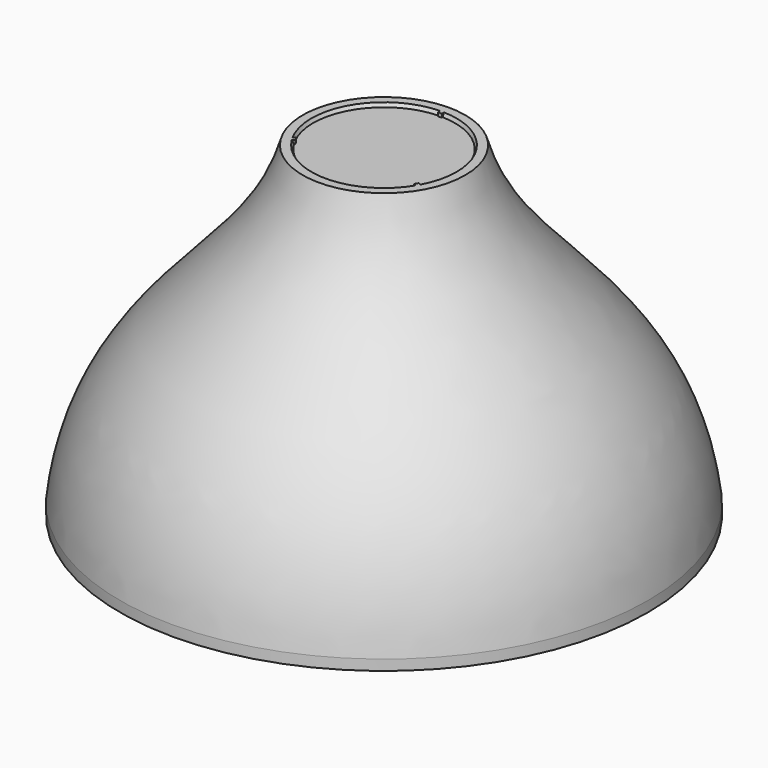
from build123d import *

# Parameters (mm, degrees)
F4_DEPTH        = 2.7018745767
F4_COPIES_COUNT = 3


# Not quite as in the source:
# - a pattern or mirror of a feature is missing from the dataset's text; its kind, count and spacing are read off the source's solid


with BuildPart() as f2:
    # F0 (on Front) → F2 (revolve)
    with BuildSketch(Plane.XZ):
        with BuildLine():
            Line((53.6962079262, 28.8167757166), (0, 28.8167757166))
            Line((0, 28.8167757166), (0, -215.1266485453))
            Line((0, -215.1266485453), (200, -215.1266485453))
            Line((200, -215.1266485453), (200, -212.5729433804))
            Line((200, -212.5729433804), (200, -207.1854621172))
            add(Edge.make_bspline(
                [(61.6075841476, 31.5186502934), (87.6578390598, -62.1243081987), (185.5585724115, -83.8800296187), (200, -207.1854621172)],
                knots=[0, 0, 0, 0, 275.9204850082, 275.9204850082, 275.9204850082, 275.9204850082], degree=3))
            Line((61.6075841476, 31.5186502934), (59, 31.5186502934))
            Line((59, 31.5186502934), (57, 31.5186502934))
            Line((57, 31.5186502934), (55, 31.5186502934))
            Line((55, 31.5186502934), (53.6962079262, 28.8167757166))
        make_face()
    revolve(axis=Axis((0, 0, -61.6418045454), (0, 0, -1)))

    # F3 (on face) → F4 (join, through all)
    with BuildSketch(Plane.XY.offset(31.5186502934)):
        Polygon((-1.5, 52.8230071068), (0, 52.8230071068), (1.5, 52.8230071068), (1.5, 55.3230071068), (0, 55.3230071068), (-1.5, 55.3230071068), align=None)
    f4 = extrude(amount=-F4_DEPTH)

    # F4_copies: F4 ×3 about axis
    f4_copies_axis = Axis((0, 0, 0), (0, 0, 1))
    for i in range(1, F4_COPIES_COUNT):
        add(f4.rotate(f4_copies_axis, i * 360 / F4_COPIES_COUNT))


solid = f2.part
